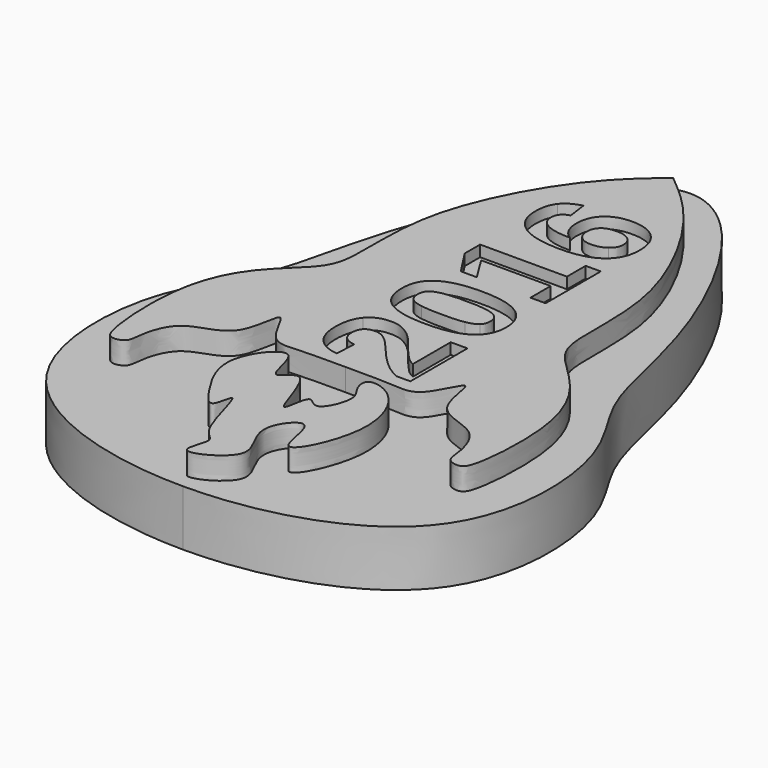
from build123d import *

# Parameters (mm, degrees)
F1_DEPTH = 6.35
F3_DEPTH = 2.54
F6_DEPTH = 2.54
F8_DEPTH = 1.27


with BuildPart() as f1:
    # F0 (on Top) → F1 (new body)
    with BuildSketch(Plane.XY):
        with BuildLine():
            Line((0, -37.4335979312), (0, 34.7609035534))
            add(Edge.make_bspline(
                [(0, 34.7609035534), (-5.9629254548, 34.7609035534), (-17.2882752808, 15.0916887633), (-18.6617189584, -1.028191267), (-26.1362359153, -9.1146428682), (-26.8026190827, -32.1015875768), (-8.9489755342, -37.4335979312), (0, -37.4335979312)],
                knots=[0, 0, 0, 0, 0.2295691522, 0.4218923762, 0.5699976771, 0.7699945744, 1, 1, 1, 1], degree=3))
        make_face()
    extrude(amount=-F1_DEPTH)

    # F2 (on face) → F3 (join)
    with BuildSketch(Plane.XY):
        with BuildLine():
            Line((0, -14.2778595909), (0, 32.3368810512))
            add(Edge.make_bspline(
                [(0, 32.3368810512), (-1.8902103034, 30.7542754081), (-6.3667619307, 27.0062791118), (-13.6090440698, 13.5446740993), (-12.3816302718, 2.6688742815), (-13.7722536243, -0.8461305318), (-18.2368273479, -4.393152646), (-21.6733100275, -11.0999933106), (-21.0024416297, -21.4423882119), (-19.9640800242, -23.035373508), (-18.1606357452, -22.6084347477), (-18.2109607569, -20.7702739722), (-16.9624841949, -16.2085739834), (-10.9066437633, -16.1842868333), (-10.9768543059, -7.9494915458), (-8.6335916035, -14.8841120259), (-5.0247985222, -14.1213720547), (-1.8953946419, -14.3746240065), (0, -14.2778595909)],
                knots=[0, 0, 0, 0, 0.0787478071, 0.1865078368, 0.2761279551, 0.3269063427, 0.3901546387, 0.4678906648, 0.5553596805, 0.5886090784, 0.6201926047, 0.6557255682, 0.7117037523, 0.7742673908, 0.8323525905, 0.8872373709, 0.9370548715, 1, 1, 1, 1], degree=3))
        make_face()
    extrude(amount=F3_DEPTH)

    # F4: F1 across face


with BuildPart() as f1_1:
    add(f1.part)
    add(f1.part.mirror(Plane(origin=(0, 0.7913483758, -2.2626194851), x_dir=(0, 1, 0), z_dir=(1, 0, 0))))

    # F5 (on face) → F6 (join)
    with BuildSketch(Plane.XY):
        with BuildLine():
            add(Edge.make_bspline(
                [(-5.4747709073, -15.6260244548), (-6.388434646, -14.9991822047), (-10.2927582675, -19.6031209003), (-7.0537341038, -24.8999573156), (-4.59238479, -28.3492970463), (-4.2161124844, -22.7283021804), (-2.5091977493, -32.1175520771), (0.058789374, -32.4554806498), (-2.5865304499, -37.1820260028), (5.6373882169, -33.0742644004), (0.1675802511, -28.6685089695), (4.8770846357, -22.8903872573), (4.8976896468, -32.7509055888), (10.076615588, -22.4223571155), (6.90561146, -15.4814357661), (2.7659757085, -14.7271587879), (3.3098080942, -17.1497077865), (4.8046016383, -18.3710986306), (2.8922193448, -22.9503870084), (0.9427506358, -19.859905444), (0.7508693233, -26.9854939454), (-1.5303223273, -15.8704358683), (-4.4535135503, -21.1496399519), (-4.636004343, -16.2014815932), (-5.4747709073, -15.6260244548)],
                knots=[0, 0, 0, 0, 0.0514922527, 0.1127508723, 0.1503874133, 0.1835871445, 0.243886854, 0.2790350101, 0.3172152466, 0.3697442186, 0.4237199156, 0.4691225826, 0.518538417, 0.5807564242, 0.6471558797, 0.6860433561, 0.7159232044, 0.7495285598, 0.7933856846, 0.8218172178, 0.8605049358, 0.9186622658, 0.9527288015, 1, 1, 1, 1], degree=3))
        make_face()
    extrude(amount=F6_DEPTH)

    # F7 (on face) → F8 (cut)
    with BuildSketch(Plane.XY.offset(2.54)):
        with BuildLine():
            add(Edge.make_bspline(
                [(6.212981767, -0.5992141387), (5.3828102258, -3.3692600761), (0.4039776837, -3.3692600761)],
                knots=[0.1667402015, 0.1667402015, 0.1667402015, 1, 1, 1], degree=2))
            Line((6.212981767, -0.5992141387), (6.212981767, 1.8448739049))
            add(Edge.make_bspline(
                [(4.8615906673, 3.6474261997), (5.8770156645, 2.9716524831), (6.212981767, 1.8448739049)],
                knots=[0, 0, 0, 0.6691374514, 0.6691374514, 0.6691374514], degree=2))
            add(Edge.make_bspline(
                [(0.4039776837, 4.6573438411), (3.3440773446, 4.6573438411), (4.8615906673, 3.6474261997)],
                knots=[0, 0, 0, 1, 1, 1], degree=2))
            add(Edge.make_bspline(
                [(-4.0800039067, 3.7014818437), (-2.5888591908, 4.6573438411), (0.4039776837, 4.6573438411)],
                knots=[0, 0, 0, 1, 1, 1], degree=2))
            add(Edge.make_bspline(
                [(-5.5711486226, 0.6862316534), (-5.5711486226, 2.7456198463), (-4.0800039067, 3.7014818437)],
                knots=[0, 0, 0, 1, 1, 1], degree=2))
            add(Edge.make_bspline(
                [(-4.9448942106, -1.6223398741), (-5.5711486226, -0.7482205578), (-5.5711486226, 0.6862316534)],
                knots=[0, 0, 0, 1, 1, 1], degree=2))
            add(Edge.make_bspline(
                [(-3.0002094573, -2.9328596332), (-4.3186397985, -2.4964591903), (-4.9448942106, -1.6223398741)],
                knots=[0, 0, 0, 1, 1, 1], degree=2))
            add(Edge.make_bspline(
                [(0.4039776837, -3.3692600761), (-1.6817791161, -3.3692600761), (-3.0002094573, -2.9328596332)],
                knots=[0, 0, 0, 1, 1, 1], degree=2))
        make_face()
        with BuildLine():
            add(Edge.make_bspline(
                [(0.4039776837, 2.3342695799), (-1.2045073326, 2.3342695799), (-2.0944478129, 2.1773763693)],
                knots=[0, 0, 0, 1, 1, 1], degree=2))
            add(Edge.make_bspline(
                [(2.8417553846, 2.1734210783), (1.9439043222, 2.3342695799), (0.4039776837, 2.3342695799)],
                knots=[0, 0, 0, 1, 1, 1], degree=2))
            add(Edge.make_bspline(
                [(4.1483198527, 1.6539595238), (3.7396064469, 2.0125725766), (2.8417553846, 2.1734210783)],
                knots=[0, 0, 0, 1, 1, 1], degree=2))
            add(Edge.make_bspline(
                [(4.5570332585, 0.6361313004), (4.5570332585, 1.295346471), (4.1483198527, 1.6539595238)],
                knots=[0, 0, 0, 1, 1, 1], degree=2))
            add(Edge.make_bspline(
                [(4.1694147382, -0.381696923), (4.5570332585, -0.0309944522), (4.5570332585, 0.6361313004)],
                knots=[0, 0, 0, 1, 1, 1], degree=2))
            add(Edge.make_bspline(
                [(2.8879004465, -0.8932478954), (3.7817962178, -0.7323993937), (4.1694147382, -0.381696923)],
                knots=[0, 0, 0, 1, 1, 1], degree=2))
            add(Edge.make_bspline(
                [(0.4039776837, -1.054096397), (1.9940046752, -1.054096397), (2.8879004465, -0.8932478954)],
                knots=[0, 0, 0, 1, 1, 1], degree=2))
            add(Edge.make_bspline(
                [(-2.0891740915, -0.9011584774), (-1.2045073326, -1.054096397), (0.4039776837, -1.054096397)],
                knots=[0, 0, 0, 1, 1, 1], degree=2))
            add(Edge.make_bspline(
                [(-3.3654146618, -0.389607505), (-2.9738408505, -0.7482205578), (-2.0891740915, -0.9011584774)],
                knots=[0, 0, 0, 1, 1, 1], degree=2))
            add(Edge.make_bspline(
                [(-3.7569884731, 0.6677736286), (-3.7569884731, -0.0309944522), (-3.3654146618, -0.389607505)],
                knots=[0, 0, 0, 1, 1, 1], degree=2))
            add(Edge.make_bspline(
                [(-3.3706883832, 1.6737359789), (-3.7569884731, 1.3269887992), (-3.7569884731, 0.6677736286)],
                knots=[0, 0, 0, 1, 1, 1], degree=2))
            add(Edge.make_bspline(
                [(-2.0944478129, 2.1773763693), (-2.9843882932, 2.0204831587), (-3.3706883832, 1.6737359789)],
                knots=[0, 0, 0, 1, 1, 1], degree=2))
        make_face(mode=Mode.SUBTRACT)
        with BuildLine():
            Line((6.212981767, 1.8448739049), (6.212981767, -0.5992141387))
            add(Edge.make_bspline(
                [(6.37910399, 0.6203101363), (6.37910399, -0.0449116048), (6.212981767, -0.5992141387)],
                knots=[0, 0, 0, 0.1667402015, 0.1667402015, 0.1667402015], degree=2))
            add(Edge.make_bspline(
                [(6.212981767, 1.8448739049), (6.37910399, 1.2877255473), (6.37910399, 0.6203101363)],
                knots=[0.6691374514, 0.6691374514, 0.6691374514, 1, 1, 1], degree=2))
        make_face()
        with BuildLine():
            Line((4.6071336114, -12.835589926), (6.212981767, -12.835589926))
            Line((6.212981767, -12.835589926), (6.212981767, -4.7114221635))
            Line((6.212981767, -4.7114221635), (4.3091683543, -4.7114221635))
            Line((4.3091683543, -4.7114221635), (4.3091683543, -10.1011653983))
            add(Edge.make_bspline(
                [(3.3045244343, -9.3958051658), (3.7738856358, -9.8691216583), (4.3091683543, -10.1011653983)],
                knots=[0, 0, 0, 1, 1, 1], degree=2))
            add(Edge.make_bspline(
                [(2.3737126134, -8.3450161838), (2.8351632329, -8.9224886733), (3.3045244343, -9.3958051658)],
                knots=[0, 0, 0, 1, 1, 1], degree=2))
            add(Edge.make_bspline(
                [(1.4257611981, -7.1544735857), (1.912261994, -7.7675436944), (2.3737126134, -8.3450161838)],
                knots=[0, 0, 0, 1, 1, 1], degree=2))
            add(Edge.make_bspline(
                [(0.3828827982, -6.0377630867), (0.9392604022, -6.5414034771), (1.4257611981, -7.1544735857)],
                knots=[0, 0, 0, 1, 1, 1], degree=2))
            add(Edge.make_bspline(
                [(-0.8327099764, -5.2137441235), (-0.1734948058, -5.5341226964), (0.3828827982, -6.0377630867)],
                knots=[0, 0, 0, 1, 1, 1], degree=2))
            add(Edge.make_bspline(
                [(-2.3067150978, -4.8933655506), (-1.491925147, -4.8933655506), (-0.8327099764, -5.2137441235)],
                knots=[0, 0, 0, 1, 1, 1], degree=2))
            add(Edge.make_bspline(
                [(-4.7141689008, -5.8980094706), (-3.8571891791, -4.8933655506), (-2.3067150978, -4.8933655506)],
                knots=[0, 0, 0, 1, 1, 1], degree=2))
            add(Edge.make_bspline(
                [(-5.5711486226, -8.7827350571), (-5.5711486226, -6.9026533906), (-4.7141689008, -5.8980094706)],
                knots=[0, 0, 0, 1, 1, 1], degree=2))
            add(Edge.make_bspline(
                [(-4.7220794829, -11.5303438882), (-5.5711486226, -10.5204262468), (-5.5711486226, -8.7827350571)],
                knots=[0, 0, 0, 1, 1, 1], degree=2))
            add(Edge.make_bspline(
                [(-2.2592516055, -12.7380260807), (-3.8730103432, -12.5402615295), (-4.7220794829, -11.5303438882)],
                knots=[0, 0, 0, 1, 1, 1], degree=2))
            Line((-2.2592516055, -12.7380260807), (-2.1274085714, -10.4044043768))
            add(Edge.make_bspline(
                [(-3.3258617516, -9.8981271258), (-2.9263773582, -10.2883825068), (-2.1274085714, -10.4044043768)],
                knots=[0, 0, 0, 1, 1, 1], degree=2))
            add(Edge.make_bspline(
                [(-3.7253461449, -8.7642770323), (-3.7253461449, -9.5078717448), (-3.3258617516, -9.8981271258)],
                knots=[0, 0, 0, 1, 1, 1], degree=2))
            add(Edge.make_bspline(
                [(-2.2091512526, -7.2401715579), (-3.7253461449, -7.2401715579), (-3.7253461449, -8.7642770323)],
                knots=[0, 0, 0, 1, 1, 1], degree=2))
            add(Edge.make_bspline(
                [(-0.947413416, -7.7306276448), (-1.5894889922, -7.2401715579), (-2.2091512526, -7.2401715579)],
                knots=[0, 0, 0, 1, 1, 1], degree=2))
            add(Edge.make_bspline(
                [(0.683484916, -9.4419502277), (-0.3053378399, -8.2210837318), (-0.947413416, -7.7306276448)],
                knots=[0, 0, 0, 1, 1, 1], degree=2))
            add(Edge.make_bspline(
                [(2.6611304278, -11.5461650523), (1.7144974428, -10.7102802159), (0.683484916, -9.4419502277)],
                knots=[0, 0, 0, 1, 1, 1], degree=2))
            add(Edge.make_bspline(
                [(4.6071336114, -12.835589926), (3.6077634128, -12.3820498886), (2.6611304278, -11.5461650523)],
                knots=[0, 0, 0, 1, 1, 1], degree=2))
        make_face()
        Polygon((4.4911117414, 6.4108561949), (6.212981767, 6.4108561949), (6.212981767, 14.2634273071), (4.4911117414, 14.2634273071), (4.4911117414, 11.6028348785), (-5.3971158176, 11.6028348785), (-5.3971158176, 9.4116036514), (-3.5117604297, 6.5031463188), (-1.6896896981, 6.5031463188), (-3.4273808878, 9.2876711994), (4.4911117414, 9.2876711994), align=None)
        with BuildLine():
            add(Edge.make_bspline(
                [(2.4132655237, 23.5082608596), (4.2669785834, 23.5082608596), (5.3230412867, 22.470656181)],
                knots=[0, 0, 0, 1, 1, 1], degree=2))
            add(Edge.make_bspline(
                [(-0.271058651, 22.6024992152), (0.7177641049, 23.5082608596), (2.4132655237, 23.5082608596)],
                knots=[0, 0, 0, 1, 1, 1], degree=2))
            add(Edge.make_bspline(
                [(-1.2598814069, 20.1383529075), (-1.2598814069, 21.6967375708), (-0.271058651, 22.6024992152)],
                knots=[0, 0, 0, 1, 1, 1], degree=2))
            add(Edge.make_bspline(
                [(-0.9302738216, 18.6458897612), (-1.2598814069, 19.3051049318), (-1.2598814069, 20.1383529075)],
                knots=[0, 0, 0, 1, 1, 1], degree=2))
            add(Edge.make_bspline(
                [(0.0163591634, 17.6175140951), (-0.6006662363, 17.9866745906), (-0.9302738216, 18.6458897612)],
                knots=[0, 0, 0, 1, 1, 1], degree=2))
            add(Edge.make_bspline(
                [(-2.8103554882, 18.1488415226), (-1.8795436673, 17.6175140951), (0.0163591634, 17.6175140951)],
                knots=[0, 0, 0, 1, 1, 1], degree=2))
            add(Edge.make_bspline(
                [(-3.741167309, 19.610980771), (-3.741167309, 18.6801689501), (-2.8103554882, 18.1488415226)],
                knots=[0, 0, 0, 1, 1, 1], degree=2))
            add(Edge.make_bspline(
                [(-2.5967697729, 21.0111537933), (-3.741167309, 20.7000042328), (-3.741167309, 19.610980771)],
                knots=[0, 0, 0, 1, 1, 1], degree=2))
            Line((-2.5967697729, 21.0111537933), (-2.9000087514, 23.1944744384))
            add(Edge.make_bspline(
                [(-4.9198440341, 21.9881106762), (-4.2685394455, 22.8411351069), (-2.9000087514, 23.1944744384)],
                knots=[0, 0, 0, 1, 1, 1], degree=2))
            add(Edge.make_bspline(
                [(-5.5711486226, 19.6610811239), (-5.5711486226, 21.1350862454), (-4.9198440341, 21.9881106762)],
                knots=[0, 0, 0, 1, 1, 1], degree=2))
            add(Edge.make_bspline(
                [(-4.0008980863, 16.4665244072), (-5.5711486226, 17.5832349062), (-5.5711486226, 19.6610811239)],
                knots=[0, 0, 0, 1, 1, 1], degree=2))
            add(Edge.make_bspline(
                [(0.675574334, 15.3498139082), (-2.4306475499, 15.3498139082), (-4.0008980863, 16.4665244072)],
                knots=[0, 0, 0, 1, 1, 1], degree=2))
            add(Edge.make_bspline(
                [(4.9406964878, 16.4507032431), (3.5022889855, 15.3498139082), (0.675574334, 15.3498139082)],
                knots=[0, 0, 0, 1, 1, 1], degree=2))
            add(Edge.make_bspline(
                [(6.37910399, 19.6030701889), (6.37910399, 17.551592578), (4.9406964878, 16.4507032431)],
                knots=[0, 0, 0, 1, 1, 1], degree=2))
            add(Edge.make_bspline(
                [(5.3230412867, 22.470656181), (6.37910399, 21.4330515025), (6.37910399, 19.6030701889)],
                knots=[0, 0, 0, 1, 1, 1], degree=2))
        make_face()
        with BuildLine():
            add(Edge.make_bspline(
                [(2.4791870407, 21.1851865984), (1.4903642848, 21.1851865984), (0.9669474394, 20.72769127)],
                knots=[0, 0, 0, 1, 1, 1], degree=2))
            add(Edge.make_bspline(
                [(4.0164768186, 20.7487861554), (3.4600992146, 21.1851865984), (2.4791870407, 21.1851865984)],
                knots=[0, 0, 0, 1, 1, 1], degree=2))
            add(Edge.make_bspline(
                [(4.5728544226, 19.5292380898), (4.5728544226, 20.3123857125), (4.0164768186, 20.7487861554)],
                knots=[0, 0, 0, 1, 1, 1], degree=2))
            add(Edge.make_bspline(
                [(3.9096839609, 18.2635449623), (4.5728544226, 18.7460904671), (4.5728544226, 19.5292380898)],
                knots=[0, 0, 0, 1, 1, 1], degree=2))
            add(Edge.make_bspline(
                [(2.2339589973, 17.7809994574), (3.2465134993, 17.7809994574), (3.9096839609, 18.2635449623)],
                knots=[0, 0, 0, 1, 1, 1], degree=2))
            add(Edge.make_bspline(
                [(0.9339866809, 18.2424500768), (1.4244427678, 17.7809994574), (2.2339589973, 17.7809994574)],
                knots=[0, 0, 0, 1, 1, 1], degree=2))
            add(Edge.make_bspline(
                [(0.4435305939, 19.4712271548), (0.4435305939, 18.7039006962), (0.9339866809, 18.2424500768)],
                knots=[0, 0, 0, 1, 1, 1], degree=2))
            add(Edge.make_bspline(
                [(0.9669474394, 20.72769127), (0.4435305939, 20.2701959416), (0.4435305939, 19.4712271548)],
                knots=[0, 0, 0, 1, 1, 1], degree=2))
        make_face(mode=Mode.SUBTRACT)
    extrude(amount=-F8_DEPTH, mode=Mode.SUBTRACT)


solid = f1_1.part
